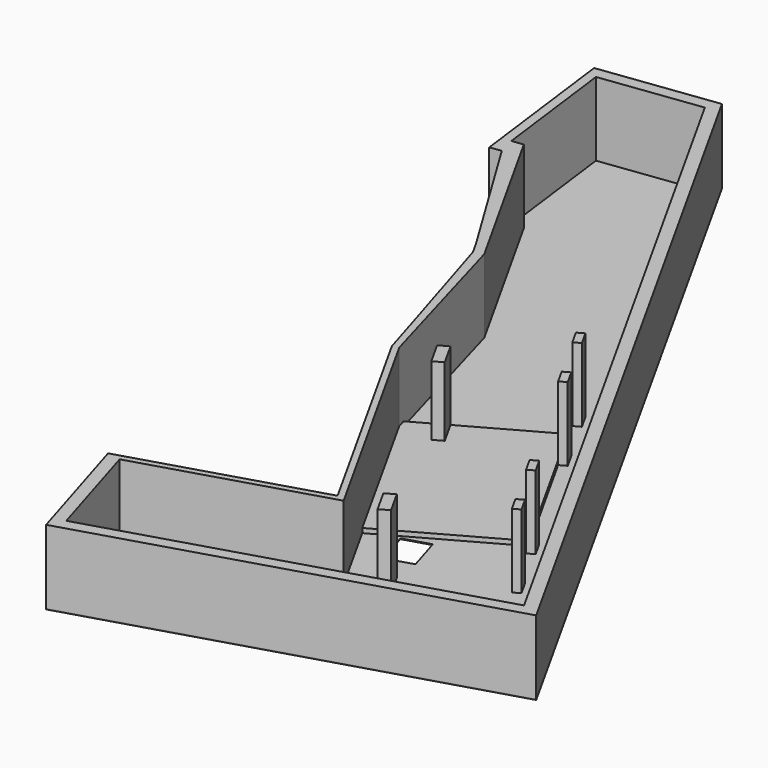
from build123d import *

# Parameters (mm, degrees)
F3_DEPTH  = 2430
F5_DEPTH  = 25
F7_DEPTH  = 2430
F9_DEPTH  = 150
F11_DEPTH = 25.001


# Not quite as in the source:
# - ends of sketch curves that miss each other by under 0.0002 mm in the source are joined


with BuildPart() as f3:
    # F2 (on Top) → F3 (new body)
    with BuildSketch(Plane.XY):
        Polygon((52902.0595629306, 50434.1230428591), (54145.32292, 46326.602018), (54431.4219269024, 46413.1983883223), (67150.915474, 50263.131268), (53075.201891, 75510.702684), (49253.5741891713, 75020.4629237414), (49304.213105, 74623.774346), (49909.660074, 69880.902321), (50281.682258, 69933.639978), (53000.597675, 65468.812402), (53225.019852, 65066.306629), (54325.972768, 61474.063518), (54760.522861, 60038.387295), (54874.022799, 59663.37285), (58991.897227, 52278.191447), (57604.002801, 51858.903346), (53909.97748, 50739.1999), align=None)
        Polygon((54412.25928, 46825.31334), (53342.81403, 50358.57026), (59287.509616, 52158.706562), (55070.827017, 59721.094989), (53523.858293, 65159.740021), (50504.389213421, 70561.8996273451), (50131.257661, 70514.151722), (49601.798244, 74661.762303), (52857.629236, 75079.514646), (66559.719817, 50502.109853), align=None, mode=Mode.SUBTRACT)
    extrude(amount=F3_DEPTH)


with BuildPart() as f5:
    # F4 (on Top) → F5 (new body)
    with BuildSketch(Plane.XY):
        Polygon((54760.522861, 60038.387295), (54874.022799, 59663.37285), (58991.897227, 52278.191447), (57604.002801, 51858.903346), (53909.97748, 50739.1999), (52902.0595629306, 50434.1230428591), (54145.32292, 46326.602018), (67150.915474, 50263.131268), (53075.201891, 75510.702684), (49253.5741891713, 75020.4629237414), (49304.213105, 74623.774346), (49909.660074, 69880.902321), (50281.682258, 69933.639978), (53000.597675, 65468.812402), (53225.019852, 65066.306629), (54325.972768, 61474.063518), align=None)
    extrude(amount=-F5_DEPTH)

    # F6 (on Top) → F7 (join)
    with BuildSketch(Plane.XY):
        Polygon((63167.175561, 54636.370609), (62899.326908, 55116.742443), (62680.976074, 54994.993056), (62948.824727, 54514.621222), align=None)
        Polygon((61606.57177, 56922.149305), (61874.420423, 56441.777471), (62092.771256, 56563.526859), (61824.922604, 57043.898693), align=None)
        Polygon((60131.75578, 53293.714353), (59826.064613, 53123.26521), (60264.362406, 52337.202212), (60570.053573, 52507.651355), align=None)
        Polygon((56498.652366, 59810.307311), (56060.354571, 60596.370312), (55754.663404, 60425.921169), (56192.961199, 59639.858168), align=None)
        Polygon((59393.320264, 61405.457583), (59174.969431, 61283.708196), (59442.818085, 60803.336359), (59661.168918, 60925.085747), align=None)
        Polygon((58586.764842, 62852.241589), (58318.916189, 63332.613423), (58100.565355, 63210.864035), (58368.414008, 62730.492201), align=None)
    extrude(amount=F7_DEPTH)

    # F10 (on face) → F11 (cut, through all)
    with BuildSketch(Plane.XY):
        Polygon((59168.735458, 53933.31513), (60028.231633, 54193.415485), (59680.654869, 55341.975624), (58821.158694, 55081.875269), align=None)
    extrude(amount=-F11_DEPTH, mode=Mode.SUBTRACT)


with BuildPart() as f9:
    # F8 (on Top) → F9 (new body)
    with BuildSketch(Plane.XY):
        Polygon((58728.797232615, 62084.088870835), (56060.354571, 60596.370312), (56498.652366, 59810.307311), (56192.961199, 59639.858168), (55754.663404, 60425.921169), (54991.3996931603, 60000.3359416475), (55070.827017, 59721.094989), (55102.8168784927, 59663.7229310719), (57874.844064254, 54692.2445670372), (58565.3824039826, 55077.2791403316), (61670.1839855803, 56808.2778988538), align=None)
    extrude(amount=F9_DEPTH)


solid = Compound([f3.part, f5.part, f9.part])
